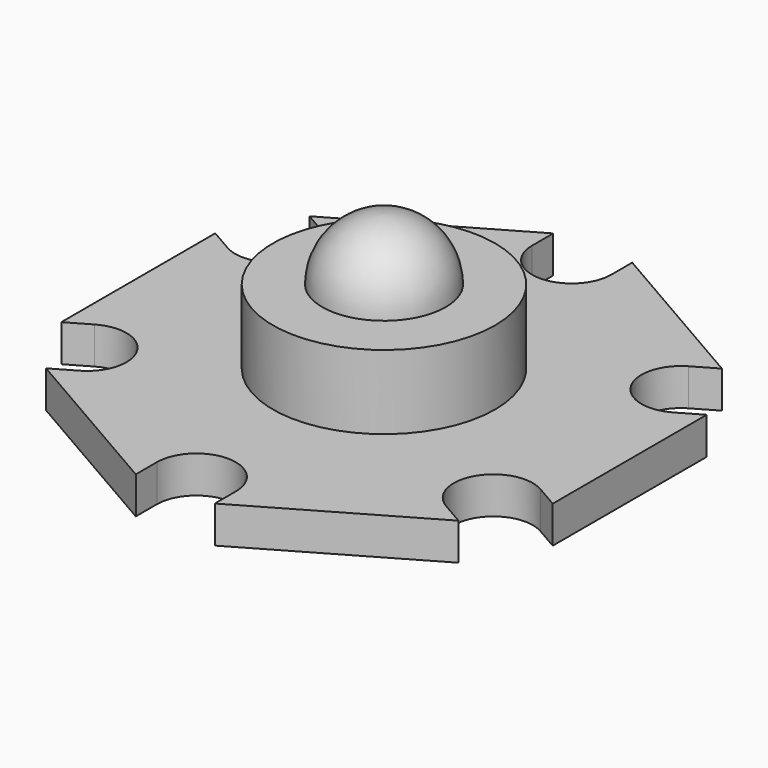
from build123d import *

# Parameters (mm, degrees)
F1_DEPTH = 1.5
F3_DEPTH = 1.501
F4_R     = 4.5
F5_DEPTH = 3
F6_R     = 2.5
F7_DEPTH = 2.5
F8_R     = 2.49999


# Not quite as in the source:
# - a fillet or chamfer is up to 0.001 mm smaller than in the source, because OpenCascade refuses the exact size


with BuildPart() as f1:
    # F0 (on Top) → F1 (new body)
    with BuildSketch(Plane.XY):
        Polygon((9.95, -5.7446351784), (9.95, 5.7446351784), (0, 11.4892703569), (-9.95, 5.7446351784), (-9.95, -5.7446351784), (0, -11.4892703569), align=None)
    extrude(amount=F1_DEPTH)

    # F2 (on face) → F3 (cut, through all)
    with BuildSketch(Plane.XY.offset(1.5)):
        with BuildLine():
            Line((-1.6, 10.5655099262), (-1.6, 9.5))
            ThreePointArc((-1.6, 9.5), (0, 7.9), (1.6, 9.5))
            Line((1.6, 9.5), (1.6, 10.5655099262))
            Line((1.6, 10.5655099262), (0, 11.4892703569))
            Line((0, 11.4892703569), (-1.6, 10.5655099262))
        make_face()
        with BuildLine():
            Line((9.95, 5.7446351784), (8.35, 6.6683956091))
            Line((8.35, 6.6683956091), (7.427241336, 6.1356406461))
            ThreePointArc((7.427241336, 6.1356406461), (6.8416006899, 3.95), (9.027241336, 3.3643593539))
            Line((9.027241336, 3.3643593539), (9.95, 3.897114317))
            Line((9.95, 3.897114317), (9.95, 5.7446351784))
        make_face()
        with BuildLine():
            Line((9.95, -5.7446351784), (9.95, -3.897114317))
            Line((9.95, -3.897114317), (9.027241336, -3.3643593539))
            ThreePointArc((9.027241336, -3.3643593539), (6.8416006899, -3.95), (7.427241336, -6.1356406461))
            Line((7.427241336, -6.1356406461), (8.35, -6.6683956091))
            Line((8.35, -6.6683956091), (9.95, -5.7446351784))
        make_face()
        with BuildLine():
            Line((-9.027241336, -3.3643593539), (-9.95, -3.897114317))
            Line((-9.95, -3.897114317), (-9.95, -5.7446351784))
            Line((-9.95, -5.7446351784), (-8.35, -6.6683956091))
            Line((-8.35, -6.6683956091), (-7.427241336, -6.1356406461))
            ThreePointArc((-7.427241336, -6.1356406461), (-6.8416006899, -3.95), (-9.027241336, -3.3643593539))
        make_face()
        with BuildLine():
            Line((-7.427241336, 6.1356406461), (-8.35, 6.6683956091))
            Line((-8.35, 6.6683956091), (-9.95, 5.7446351784))
            Line((-9.95, 5.7446351784), (-9.95, 3.897114317))
            Line((-9.95, 3.897114317), (-9.027241336, 3.3643593539))
            ThreePointArc((-9.027241336, 3.3643593539), (-6.8416006899, 3.95), (-7.427241336, 6.1356406461))
        make_face()
        with BuildLine():
            Line((-1.6, -9.5), (-1.6, -10.5655099262))
            Line((-1.6, -10.5655099262), (0, -11.4892703569))
            Line((0, -11.4892703569), (1.6, -10.5655099262))
            Line((1.6, -10.5655099262), (1.6, -9.5))
            ThreePointArc((1.6, -9.5), (0, -7.9), (-1.6, -9.5))
        make_face()
    extrude(amount=-F3_DEPTH, mode=Mode.SUBTRACT)

    # F4 (on face) → F5 (join)
    with BuildSketch(Plane.XY.offset(1.5)):
        Circle(F4_R)
    extrude(amount=F5_DEPTH)

    # F6 (on face) → F7 (join)
    with BuildSketch(Plane.XY.offset(4.5)):
        Circle(F6_R)
    extrude(amount=F7_DEPTH)

    # F8 (radius 2.5 in the source; OpenCascade refuses exactly that, so slightly less here)
    f8_edges = [f1.edges().sort_by_distance(p)[0] for p in [
        (-2.5, 0, 7),
    ]]
    fillet(f8_edges, radius=F8_R)


solid = f1.part
